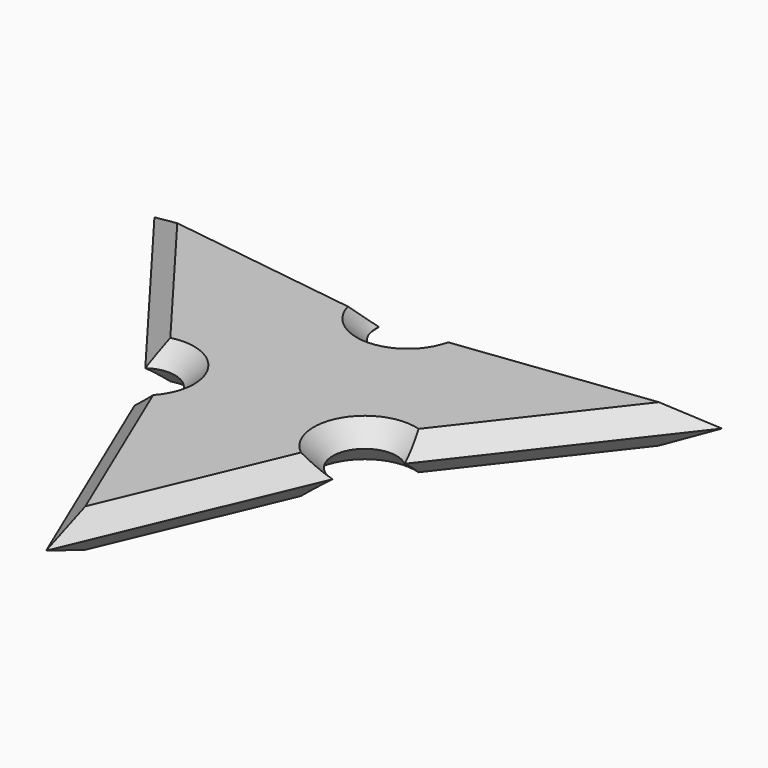
from build123d import *

# Parameters (mm, degrees)
F1_DEPTH = 7.62
F2_SIZE  = 3.81
F3_SIZE  = 3.80999


# Not quite as in the source:
# - a fillet or chamfer is up to 0.001 mm smaller than in the source, because OpenCascade refuses the exact size
# - a feature names something its author has since deleted; it is built from what else it names


with BuildPart() as f1:
    # F0 (on Top) → F1 (new body)
    with BuildSketch(Plane.XY):
        with BuildLine():
            Line((-20.2860954264, -4.4913191196), (-0.4820694779, -51.2720903428))
            Line((-0.4820694779, -51.2720903428), (19.2434711163, -4.6767160388))
            ThreePointArc((19.2434711163, -4.6767160388), (15.0404138493, 4.3253448413), (24.7550324356, 6.4059640289))
            Line((24.7550324356, 6.4059640289), (55.8461389062, 46.4629190132))
            Line((55.8461389062, 46.4629190132), (5.4307896441, 40.2233229702))
            ThreePointArc((5.4307896441, 40.2233229702), (-0.645142483, 32.7880593977), (-7.1331060464, 39.8666485513))
            Line((-7.1331060464, 39.8666485513), (-57.4455202297, 46.8881141422))
            Line((-57.4455202297, 46.8881141422), (-26.8341969161, 6.3469389621))
            ThreePointArc((-26.8341969161, 6.3469389621), (-17.7091606963, 4.4627734196), (-20.2860954264, -4.4913191196))
        make_face()
    extrude(amount=F1_DEPTH)

    # F2
    f2_edges = [f1.edges().sort_by_distance(p)[0] for p in [
        (-32.289313, 43.377381, 0),
        (30.638464, 43.343121, 0),
        (-42.139859, 26.617527, 0),
        (40.300586, 26.434442, 0),
        (9.380701, -27.974403, 0),
        (-10.384082, -27.881705, 0),
        (15.040414, 4.325345, 0),
    ]]
    chamfer(f2_edges, length=F2_SIZE)

    # F3 (size 3.81 in the source; OpenCascade refuses exactly that, so slightly less here)
    f3_edges = [f1.edges().sort_by_distance(p)[0] for p in [
        (-32.289313, 43.377381, 7.62),
        (-42.139859, 26.617527, 7.62),
        (-10.384082, -27.881705, 7.62),
        (9.380701, -27.974403, 7.62),
        (40.300586, 26.434442, 7.62),
        (30.638464, 43.343121, 7.62),
        (15.040414, 4.325345, 7.62),
        (-0.645142, 32.788059, 7.62),
        (-17.709161, 4.462773, 7.62),
        (-17.729481, 4.496175, 0),
        (-0.591, 32.789828, 0),
    ]]
    chamfer(f3_edges, length=F3_SIZE)


solid = f1.part
